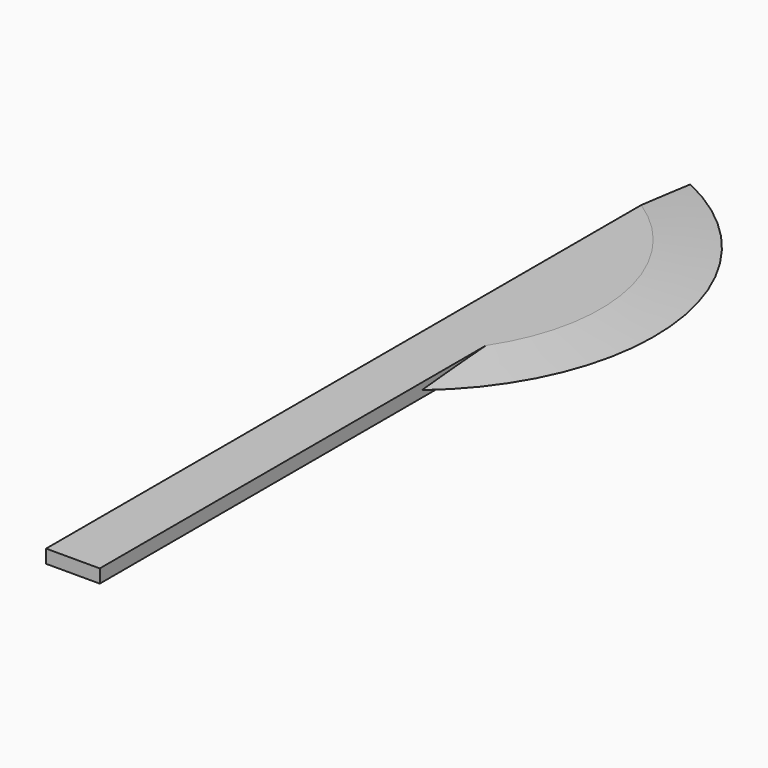
from build123d import *

# Parameters (mm, degrees)
F1_DEPTH = 1.27
F2_SIZE2 = 0.635
F2_SIZE  = 5.08
F3_SIZE2 = 5.07999
F3_SIZE  = 0.63499


# Not quite as in the source:
# - a fillet or chamfer is up to 0.001 mm smaller than in the source, because OpenCascade refuses the exact size


with BuildPart() as f1:
    # F0 (on Top) → F1 (new body)
    with BuildSketch(Plane.XY):
        with BuildLine():
            Line((-36.8330654015, 25.4), (-36.8330654015, 0))
            Line((-36.8330654015, 0), (-31.7530654015, 0))
            Line((-31.7530654015, 0), (-31.7530654015, 25.4))
            Line((-31.7530654015, 25.4), (-31.7530654015, 38.1))
            ThreePointArc((-31.7530654015, 38.1), (-23.9034396028, 58.5352834398), (-36.8330654015, 76.2))
            Line((-36.8330654015, 76.2), (-36.8330654015, 25.4))
        make_face()
    extrude(amount=F1_DEPTH)

    # F2
    f2_edges = [f1.edges().sort_by_distance(p)[0] for p in [
        (-23.90344, 58.535283, 1.27),
    ]]
    f2_side = f1.faces().sort_by_distance((-32.33426, 43.519124, 1.27))[0]
    chamfer(f2_edges, length=F2_SIZE, length2=F2_SIZE2, reference=f2_side)

    # F3 (size 0.635 and 5.08 in the source; OpenCascade refuses exactly that, so slightly less here)
    f3_edges = [f1.edges().sort_by_distance(p)[0] for p in [
        (-23.90344, 58.535283, 0),
    ]]
    f3_side = f1.faces().sort_by_distance((-23.90344, 58.535283, 0.3175))[0]
    chamfer(f3_edges, length=F3_SIZE, length2=F3_SIZE2, reference=f3_side)


solid = f1.part
